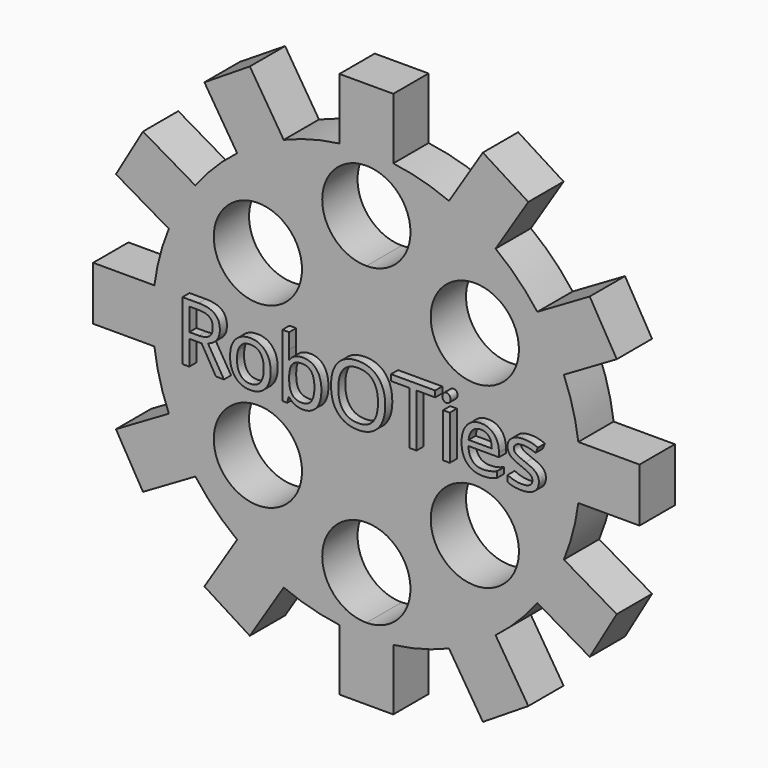
from build123d import *

# Parameters (mm, degrees)
F1_DEPTH     = 12.7
F2_R         = 12.7
F3_DEPTH     = 25.4
F4_TEXT_SIZE = 23.7779643586
F5_DEPTH     = 2.54


# Not quite as in the source:
# - Text() gives the source's letters only with a copy of the font that has no kerning and outlines rounded to 1/6400 em; it was checked with that copy


with BuildPart() as f1:
    # F0 (on Front) → F1 (new body)
    with BuildSketch(Plane.XZ):
        with BuildLine():
            ThreePointArc((-56.8500334606, 23.4278029543), (-59.4450508004, 15.7185938008), (-60.9997447474, 7.7343))
            Line((-60.9997447474, 7.7343), (-78.6273447474, 7.7343))
            Line((-78.6273447474, 7.7343), (-78.6273447474, 0))
            Line((-78.6273447474, 0), (-78.6273447474, -7.7343))
            Line((-78.6273447474, -7.7343), (-60.9997447474, -7.7343))
            ThreePointArc((-60.9997447474, -7.7343), (-59.4450508004, -15.7185938008), (-56.8500334606, -23.4278029543))
            Line((-56.8500334606, -23.4278029543), (-72.0703548158, -32.3006127958))
            Line((-72.0703548158, -32.3006127958), (-64.2848588429, -45.6557677844))
            Line((-64.2848588429, -45.6557677844), (-49.2095239655, -36.8674789866))
            ThreePointArc((-49.2095239655, -36.8674789866), (-43.6224896133, -43.3343588354), (-37.1927765408, -48.9641259385))
            Line((-37.1927765408, -48.9641259385), (-46.6130534616, -63.863477082))
            Line((-46.6130534616, -63.863477082), (-33.5385508011, -72.1299736882))
            Line((-33.5385508011, -72.1299736882), (-23.7840050246, -56.701934365))
            ThreePointArc((-23.7840050246, -56.701934365), (-15.9111721896, -59.3937947541), (-7.747, -60.9981331414))
            Line((-7.747, -60.9981331414), (-7.747, -78.6257331414))
            Line((-7.747, -78.6257331414), (0, -78.6257331414))
            Line((0, -78.6257331414), (7.747, -78.6257331414))
            Line((7.747, -78.6257331414), (7.747, -60.9981331414))
            ThreePointArc((7.747, -60.9981331414), (15.9111721896, -59.3937947541), (23.7840050246, -56.701934365))
            Line((23.7840050246, -56.701934365), (33.5385508011, -72.1299736882))
            Line((33.5385508011, -72.1299736882), (46.6130534616, -63.863477082))
            Line((46.6130534616, -63.863477082), (37.1927765408, -48.9641259385))
            ThreePointArc((37.1927765408, -48.9641259385), (43.6224896133, -43.3343588354), (49.2095239655, -36.8674789866))
            Line((49.2095239655, -36.8674789866), (64.2848588429, -45.6557677844))
            Line((64.2848588429, -45.6557677844), (72.0703548158, -32.3006127958))
            Line((72.0703548158, -32.3006127958), (56.8500334606, -23.4278029543))
            ThreePointArc((56.8500334606, -23.4278029543), (59.4450508004, -15.7185938008), (60.9997447474, -7.7343))
            Line((60.9997447474, -7.7343), (78.6273447474, -7.7343))
            Line((78.6273447474, -7.7343), (78.6273447474, 0))
            Line((78.6273447474, 0), (78.6273447474, 7.7343))
            Line((78.6273447474, 7.7343), (60.9997447474, 7.7343))
            ThreePointArc((60.9997447474, 7.7343), (59.4450508004, 15.7185938008), (56.8500334606, 23.4278029543))
            Line((56.8500334606, 23.4278029543), (72.0703548158, 32.3006127958))
            Line((72.0703548158, 32.3006127958), (64.2848588429, 45.6557677844))
            Line((64.2848588429, 45.6557677844), (49.2095239655, 36.8674789866))
            ThreePointArc((49.2095239655, 36.8674789866), (43.6224896133, 43.3343588354), (37.1927765408, 48.9641259385))
            Line((37.1927765408, 48.9641259385), (46.6130534616, 63.863477082))
            Line((46.6130534616, 63.863477082), (33.5385508011, 72.1299736882))
            Line((33.5385508011, 72.1299736882), (23.7840050246, 56.701934365))
            ThreePointArc((23.7840050246, 56.701934365), (15.9111721896, 59.3937947541), (7.747, 60.9981331414))
            Line((7.747, 60.9981331414), (7.747, 78.6257331414))
            Line((7.747, 78.6257331414), (0, 78.6257331414))
            Line((0, 78.6257331414), (-7.747, 78.6257331414))
            Line((-7.747, 78.6257331414), (-7.747, 60.9981331414))
            ThreePointArc((-7.747, 60.9981331414), (-15.9111721896, 59.3937947541), (-23.7840050246, 56.701934365))
            Line((-23.7840050246, 56.701934365), (-33.5385508011, 72.1299736882))
            Line((-33.5385508011, 72.1299736882), (-46.6130534616, 63.863477082))
            Line((-46.6130534616, 63.863477082), (-37.1927765408, 48.9641259385))
            ThreePointArc((-37.1927765408, 48.9641259385), (-43.6224896133, 43.3343588354), (-49.2095239655, 36.8674789866))
            Line((-49.2095239655, 36.8674789866), (-64.2848588429, 45.6557677844))
            Line((-64.2848588429, 45.6557677844), (-72.0703548158, 32.3006127958))
            Line((-72.0703548158, 32.3006127958), (-56.8500334606, 23.4278029543))
        make_face()
    extrude(amount=F1_DEPTH)

    # F2 (on face) → F3 (cut)
    with BuildSketch(Plane.XZ.offset(12.7)):
        with Locations((-31.2176030129, 25.6263930351)):
            Circle(F2_R)
        with BuildLine():
            ThreePointArc((0, 32.4956354082), (12.6999994745, 45.1956354082), (0, 57.8956354082))
            ThreePointArc((0, 57.8956354082), (-12.6999994745, 45.1956354082), (0, 32.4956354082))
        make_face()
        with Locations((31.2176030129, 25.6263930351)):
            Circle(F2_R)
        with Locations((-31.2176030129, -25.6263930351)):
            Circle(F2_R)
        with BuildLine():
            ThreePointArc((0, -32.4956354082), (-12.6999994745, -45.1956354082), (0, -57.8956354082))
            ThreePointArc((0, -57.8956354082), (12.6999994745, -45.1956354082), (0, -32.4956354082))
        make_face()
        with Locations((31.2176030129, -25.6263930351)):
            Circle(F2_R)
    extrude(amount=-F3_DEPTH, mode=Mode.SUBTRACT)

    # F4 (on face) → F5 (join)
    with BuildSketch(Plane.XZ.offset(12.7)):
        with Locations((-53.2273447474, -7.898670755)):
            Text('RobOTies', F4_TEXT_SIZE, font='Open Sans', text_align=(TextAlign.LEFT, TextAlign.BOTTOM))
    extrude(amount=F5_DEPTH)


solid = f1.part
